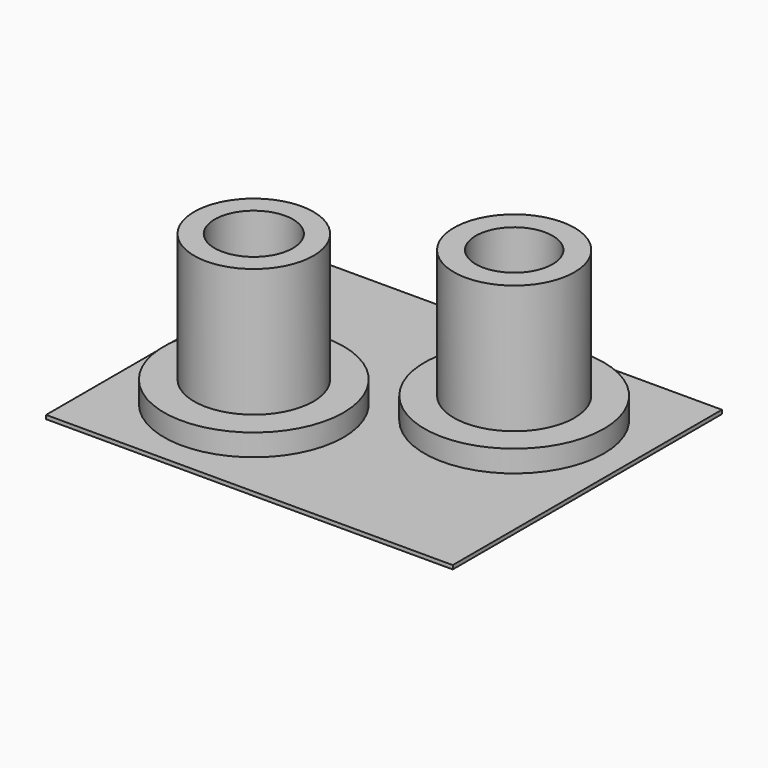
from build123d import *

# Parameters (mm, degrees)
F0_R     = 7
F0_R_2   = 4.7
F0_R_3   = 3
F1_DEPTH = 2
F2_DEPTH = 12
F0_R_4   = 4.65
F3_DEPTH = 2
F0_R_5   = 3.05
F4_DEPTH = 12
F0_W     = 31.71593739
F0_H     = 26.2385108796
F5_DEPTH = 0.3


with BuildPart() as f1:
    # F0 (on Top) → F1 (new body)
    with BuildSketch(Plane.XY):
        Circle(F0_R)
        Circle(F0_R_2, mode=Mode.SUBTRACT)
        Circle(F0_R_2)
        Circle(F0_R_3, mode=Mode.SUBTRACT)
    extrude(amount=F1_DEPTH)

    # F0 (on Top) → F2 (join)
    with BuildSketch(Plane.XY):
        Circle(F0_R_2)
        Circle(F0_R_3, mode=Mode.SUBTRACT)
    extrude(amount=F2_DEPTH)



with BuildPart() as f3:
    # F0 (on Top) → F3 (new body)
    with BuildSketch(Plane.XY):
        with Locations((-13.71593739, -8.2385108796)):
            Circle(F0_R)
        with Locations((-13.71593739, -8.2385108796)):
            Circle(F0_R_4, mode=Mode.SUBTRACT)
    extrude(amount=F3_DEPTH)

    # F0 (on Top) → F4 (join)
    with BuildSketch(Plane.XY):
        with Locations((-13.71593739, -8.2385108796)):
            Circle(F0_R_4)
        with Locations((-13.71593739, -8.2385108796)):
            Circle(F0_R_5, mode=Mode.SUBTRACT)
    extrude(amount=F4_DEPTH)


with BuildPart() as f1_1:
    add(f1.part)

    add(f3.part)  # F5 merges F3
    # F0 (on Top) → F5 (join)
    with BuildSketch(Plane.XY):
        with Locations((-6.857968695, -4.1192554398)):
            Rectangle(F0_W, F0_H)
        with Locations((-13.71593739, -8.2385108796)):
            Circle(F0_R, mode=Mode.SUBTRACT)
        Circle(F0_R, mode=Mode.SUBTRACT)
        with Locations((-13.71593739, -8.2385108796)):
            Circle(F0_R)
        with Locations((-13.71593739, -8.2385108796)):
            Circle(F0_R_4, mode=Mode.SUBTRACT)
        Circle(F0_R)
        Circle(F0_R_2, mode=Mode.SUBTRACT)
        Circle(F0_R_2)
        Circle(F0_R_3, mode=Mode.SUBTRACT)
        with Locations((-13.71593739, -8.2385108796)):
            Circle(F0_R_4)
        with Locations((-13.71593739, -8.2385108796)):
            Circle(F0_R_5, mode=Mode.SUBTRACT)
        with Locations((-13.71593739, -8.2385108796)):
            Circle(F0_R_5)
        Circle(F0_R_3)
    extrude(amount=F5_DEPTH)


solid = f1_1.part
